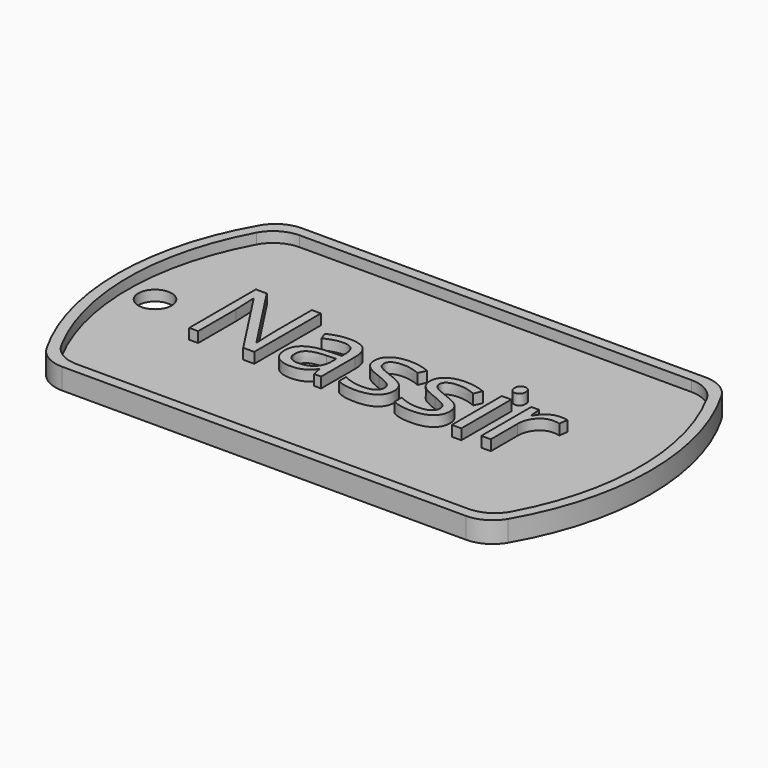
from build123d import *

# Parameters (mm, degrees)
F1_DEPTH     = 1
F3_DEPTH     = 1
F4_R         = 1.5875
F5_DEPTH     = 1
F6_TEXT_SIZE = 11.1139130442
F7_DEPTH     = 1


# Not quite as in the source:
# - Text() gives the source's letters only with a copy of the font that has no kerning and outlines rounded to 1/6400 em; it was checked with that copy


with BuildPart() as f1:
    # F0 (on Top) → F1 (new body)
    with BuildSketch(Plane.XY):
        with BuildLine():
            ThreePointArc((-19.2474145991, 14.2875), (-20.8349145991, 13.862130657), (-21.9970452561, 12.7))
            ThreePointArc((-21.9970452561, 12.7), (-25.4, 0), (-21.9970452561, -12.7))
            ThreePointArc((-21.9970452561, -12.7), (-20.8349145991, -13.862130657), (-19.2474145991, -14.2875))
            Line((-19.2474145991, -14.2875), (19.2474145991, -14.2875))
            ThreePointArc((19.2474145991, -14.2875), (20.8349145991, -13.862130657), (21.9970452561, -12.7))
            ThreePointArc((21.9970452561, -12.7), (25.4, 0), (21.9970452561, 12.7))
            ThreePointArc((21.9970452561, 12.7), (20.8349145991, 13.862130657), (19.2474145991, 14.2875))
            Line((19.2474145991, 14.2875), (-19.2474145991, 14.2875))
        make_face()
    extrude(amount=F1_DEPTH)

    # F2 (on face) → F3 (join)
    with BuildSketch(Plane.XY.offset(1)):
        with BuildLine():
            Line((19.2474145991, 14.2875), (-19.2474145991, 14.2875))
            ThreePointArc((-19.2474145991, 14.2875), (-20.8349145991, 13.862130657), (-21.9970452561, 12.7))
            ThreePointArc((-21.9970452561, 12.7), (-25.4, 0), (-21.9970452561, -12.7))
            ThreePointArc((-21.9970452561, -12.7), (-20.8349145991, -13.862130657), (-19.2474145991, -14.2875))
            Line((-19.2474145991, -14.2875), (19.2474145991, -14.2875))
            ThreePointArc((19.2474145991, -14.2875), (20.8349145991, -13.862130657), (21.9970452561, -12.7))
            ThreePointArc((21.9970452561, -12.7), (25.4, 0), (21.9970452561, 12.7))
            ThreePointArc((21.9970452561, 12.7), (20.8349145991, 13.862130657), (19.2474145991, 14.2875))
        make_face()
        with BuildLine():
            ThreePointArc((-21.4526124879, 11.6252061249), (-20.2856017842, 12.8404540819), (-18.6611352482, 13.2875))
            Line((-18.6611352482, 13.2875), (18.6611352482, 13.2875))
            ThreePointArc((18.6611352482, 13.2875), (20.2856017842, 12.8404540819), (21.4526124879, 11.6252061249))
            ThreePointArc((21.4526124879, 11.6252061249), (24.4, 0), (21.4526124879, -11.6252061249))
            ThreePointArc((21.4526124879, -11.6252061249), (20.2856017842, -12.8404540819), (18.6611352482, -13.2875))
            Line((18.6611352482, -13.2875), (-18.6611352482, -13.2875))
            ThreePointArc((-18.6611352482, -13.2875), (-20.2856017842, -12.8404540819), (-21.4526124879, -11.6252061249))
            ThreePointArc((-21.4526124879, -11.6252061249), (-24.4, 0), (-21.4526124879, 11.6252061249))
        make_face(mode=Mode.SUBTRACT)
    extrude(amount=F3_DEPTH)

    # F4 (on face) → F5 (cut)
    with BuildSketch(Plane.XY.offset(1)):
        with Locations((-21.821282804, 0)):
            Circle(F4_R)
    extrude(amount=-F5_DEPTH, mode=Mode.SUBTRACT)

    # F6 (on face) → F7 (join)
    with BuildSketch(Plane.XY.offset(1)):
        with Locations((-16.8608035892, -3.4879038576)):
            Text('Nassir', F6_TEXT_SIZE, font='Open Sans', text_align=(TextAlign.LEFT, TextAlign.BOTTOM))
    extrude(amount=F7_DEPTH)


solid = f1.part
